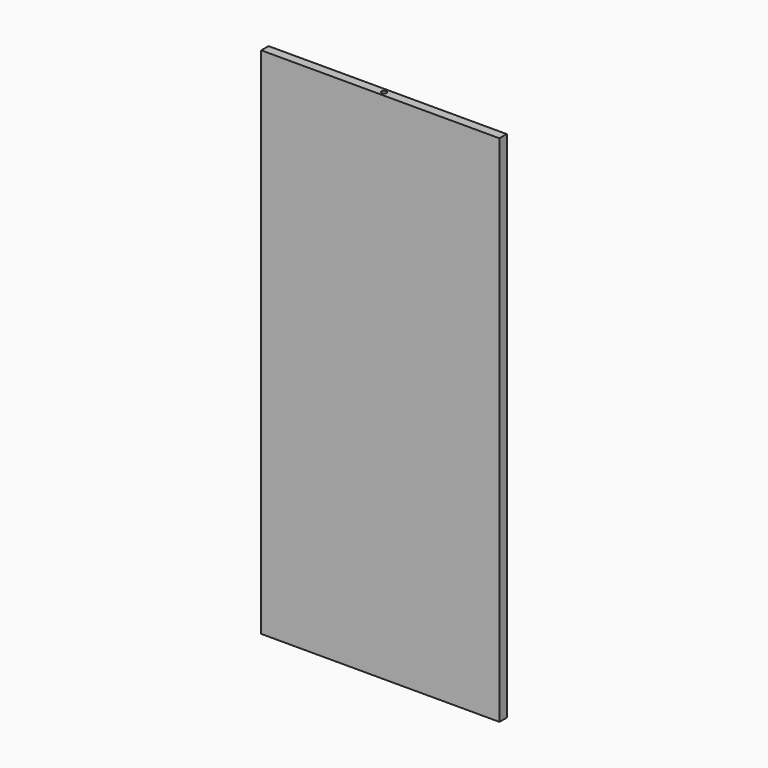
from build123d import *

# Parameters (mm, degrees)
F0_W     = 165.0993153453
F0_H     = 356.130450964
F1_DEPTH = 6.35
F3_D     = 3.4544
F3_DEPTH = 18.25625
F3_TIP   = 1.0378064612


# Not quite as in the source:
# - a length typed as a fraction of an inch, garbled in the dataset ("3 / 203.2 mm" for 3/8 in), is restored


with BuildPart() as f1:
    # F0 (on Front) → F1 (new body)
    with BuildSketch(Plane.XZ):
        with Locations((-14.4004262984, -14.0939205885)):
            Rectangle(F0_W, F0_H)
    extrude(amount=F1_DEPTH)

    # F3
    with Locations(Plane.XY.offset(163.9713048935)):
        with Locations((-14.4004262984, -3.175)):
            Hole(F3_D / 2, depth=F3_DEPTH)
            with Locations((0, 0, -(F3_DEPTH + F3_TIP / 2))):  # 118° drill point
                Cone(0, F3_D / 2, F3_TIP, mode=Mode.SUBTRACT)


solid = f1.part
